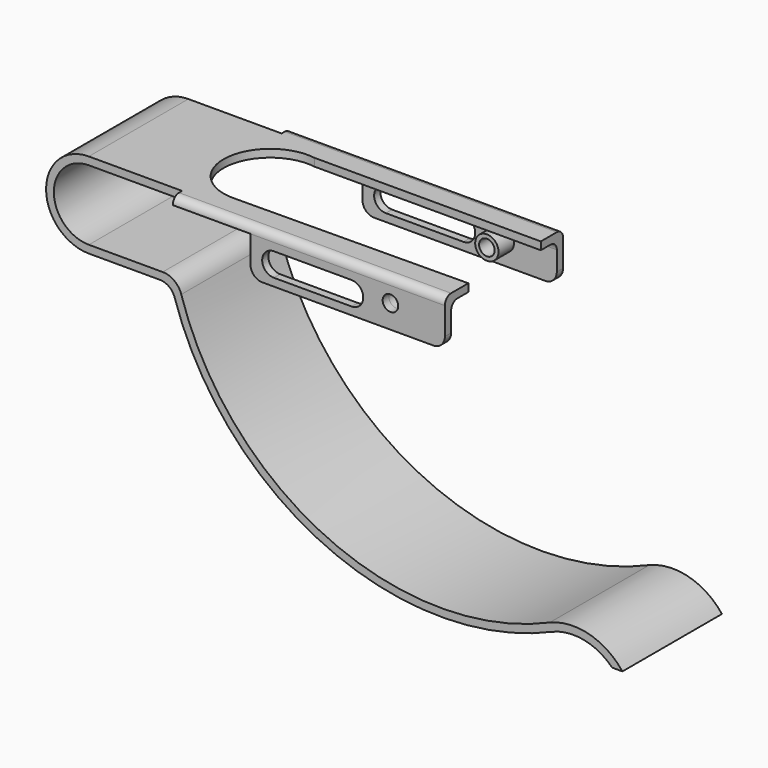
from build123d import *

# Parameters (mm, degrees)
F1_DEPTH  = 16
F2_W      = 70
F2_H      = 3
F3_DEPTH  = 2
F4_W      = 50
F4_H      = 12
F5_DEPTH  = 2
F6_R      = 2
F9_DEPTH  = 2
F11_DEPTH = 38.001
F13_D     = 4
F14_R     = 3
F14_R_2   = 2
F15_DEPTH = 5
F16_R     = 3


# Not quite as in the source:
# - a pattern or mirror of a feature is missing from the dataset's text; its kind, count and spacing are read off the source's solid


with BuildPart() as f1:
    # F0 (on Front) → F1 (new body)
    with BuildSketch(Plane.XZ):
        with BuildLine():
            ThreePointArc((0, -9), (-9, 0), (0, 9))
            Line((0, 9), (94, 9))
            Line((94, 9), (94, 11))
            Line((94, 11), (0, 11))
            ThreePointArc((0, 11), (-11, 0), (0, -11))
            Line((0, -11), (18.2665281953, -11))
            ThreePointArc((18.2665281953, -11), (20.6244584971, -11.7688756304), (22.0759112253, -13.779917654))
            ThreePointArc((22.0759112253, -13.779917654), (60.9393672504, -57.4049197249), (119.3629664678, -57.8431826489))
            ThreePointArc((119.3629664678, -57.8431826489), (127.4740086729, -57.1014451531), (134.6252638265, -61))
            Line((134.6252638265, -61), (137.2771081943, -61))
            ThreePointArc((137.2771081943, -61), (128.7730913255, -55.3547464626), (118.5862940723, -56))
            ThreePointArc((118.5862940723, -56), (61.4655553189, -55.4468201567), (23.7763203843, -12.5212290284))
            ThreePointArc((23.7763203843, -12.5212290284), (21.9669972314, -9.9754593518), (19, -9))
            Line((19, -9), (0, -9))
        make_face()
    extrude(amount=F1_DEPTH)

    # F2 (on face) → F3 (join)
    with BuildSketch(Plane.XY.offset(11)):
        with Locations((59, -17.5)):
            Rectangle(F2_W, F2_H)
    extrude(amount=-F3_DEPTH)

    # F4 (on face) → F5 (join)
    with BuildSketch(Plane.XZ.offset(19)):
        with Locations((69, 5)):
            Rectangle(F4_W, F4_H)
    extrude(amount=-F5_DEPTH)

    # F6
    f6_edges = [f1.edges().sort_by_distance(p)[0] for p in [
        (59, -19, 11),
        (69, -17, 9),
    ]]
    fillet(f6_edges, radius=F6_R)

    # F7: F1 across plane


with BuildPart() as f1_1:
    add(f1.part)
    add(f1.part.mirror(Plane.XZ))

    # F8 (on face) → F9 (cut)
    with BuildSketch(Plane.XY.offset(11)):
        with BuildLine():
            Line((94, 11.8473697647), (35.7999188125, 11.8473697647))
            ThreePointArc((35.7999188125, 11.8473697647), (21.9261214029, 0.9031688421), (34, -11.9995147554))
            Line((34, -11.9995147554), (94, -11.4599181938))
            Line((94, -11.4599181938), (94, 11.8473697647))
        make_face()
    extrude(amount=-F9_DEPTH, mode=Mode.SUBTRACT)

    # F10 (on face) → F11 (cut, through all)
    with BuildSketch(Plane.XZ.offset(19)):
        with BuildLine():
            ThreePointArc((50, 7), (47, 4), (50, 1))
            Line((50, 1), (70, 1))
            ThreePointArc((70, 1), (73, 4), (70, 7))
            Line((70, 7), (50, 7))
        make_face()
    extrude(amount=-F11_DEPTH, mode=Mode.SUBTRACT)

    # F13 (through all)
    with Locations(Plane.XZ.offset(19)):
        with Locations((80, 5)):
            Hole(F13_D / 2)

    # F14 (on face) → F15 (join)
    with BuildSketch(Plane(origin=(0, -17, 0), x_dir=(-1, 0, 0), z_dir=(0, 1, 0))):
        with Locations((-80, 5)):
            Circle(F14_R)
        with Locations((-80, 5)):
            Circle(F14_R_2, mode=Mode.SUBTRACT)
    f15 = extrude(amount=F15_DEPTH)

    # F15_copies: F15 across plane
    add(f15.mirror(Plane.ZX))

    # F16
    f16_edges = [f1_1.edges().sort_by_distance(p)[0] for p in [
        (94, -18, -1),
        (94, 18, -1),
        (44, 18, -1),
        (44, -18, -1),
    ]]
    fillet(f16_edges, radius=F16_R)


solid = f1_1.part
